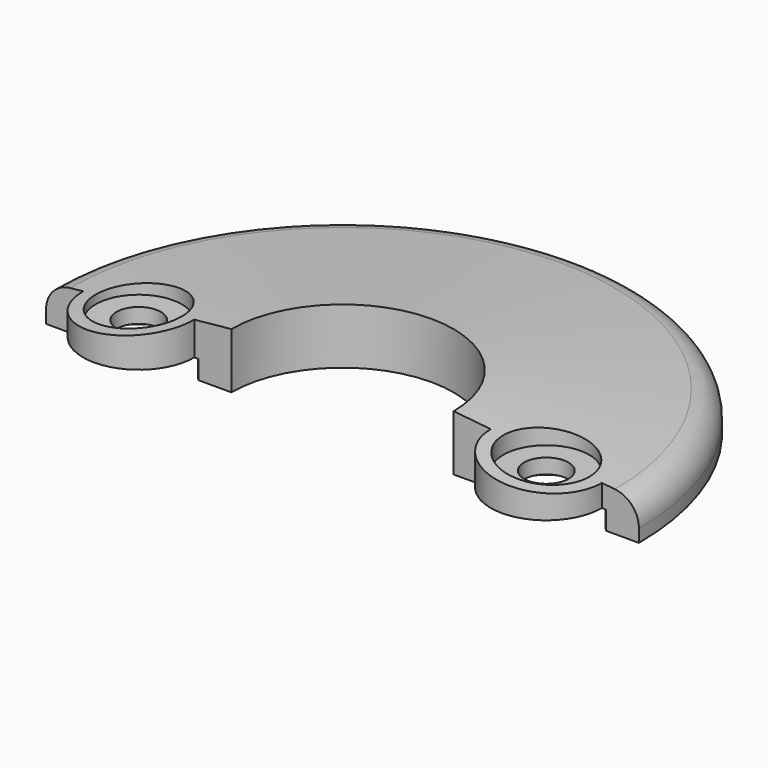
from build123d import *

# Parameters (mm, degrees)
F3_DEPTH     = 4.7762
F4_R         = 4.8895
F5_DEPTH     = 1.6002
F6_R         = 1.905
F7_DEPTH     = 3.1760001
F9_R         = 3.683
F10_DEPTH    = 1.9060001
F11_T1_DEPTH = 2.2381504403


# Not quite as in the source:
# - a fillet or chamfer that OpenCascade refuses, or shapes differently, is made with other operations: its cross-section is extruded or revolved along the edge and cut away or added


with BuildPart() as f1:
    # F0 (on Front) → F1 (revolve)
    with BuildSketch(Plane.XZ):
        with BuildLine():
            Line((9.525, 4.7752), (9.525, 0))
            Line((9.525, 0), (25.4, 0))
            Line((25.4, 0), (25.4, 1.10784454))
            ThreePointArc((25.4, 1.10784454), (24.8095678029, 2.6410913648), (23.343266994, 3.382318687))
            Line((23.343266994, 3.382318687), (9.525, 4.7752))
        make_face()
    revolve(axis=Axis((0, 0, 2.1961550228), (0, 0, 1)))

    # F2 (on face) → F3 (cut, through all)
    with BuildSketch(Plane(origin=(0, 0, 0), x_dir=(1, 0, 0), z_dir=(0, 0, -1))):
        with BuildLine():
            Line((-25.4, 25.4), (-25.4, 0))
            Line((-25.4, 0), (-22.225, 0))
            ThreePointArc((-22.225, 0), (-17.4625, 4.7625), (-12.7, 0))
            Line((-12.7, 0), (-9.525, 0))
            ThreePointArc((-9.525, 0), (0, 9.525), (9.525, 0))
            Line((9.525, 0), (12.7, 0))
            ThreePointArc((12.7, 0), (17.4625, 4.7625), (22.225, 0))
            Line((22.225, 0), (25.4, 0))
            Line((25.4, 0), (25.4, 25.4))
            Line((25.4, 25.4), (-25.4, 25.4))
        make_face()
        with BuildLine():
            ThreePointArc((9.525, 0), (0, 9.525), (-9.525, 0))
            ThreePointArc((-9.525, 0), (0, -9.525), (9.525, 0))
        make_face()
    extrude(amount=-F3_DEPTH, mode=Mode.SUBTRACT)

    # F4 (on face) → F5 (cut)
    with BuildSketch(Plane(origin=(0, 0, 0), x_dir=(1, 0, 0), z_dir=(0, 0, -1))):
        with Locations((-17.4625, 0)):
            Circle(F4_R)
        with Locations((17.4625, 0)):
            Circle(F4_R)
    extrude(amount=-F5_DEPTH, mode=Mode.SUBTRACT)

    # F6 (on face) → F7 (cut, through all)
    with BuildSketch(Plane(origin=(0, 0, 1.6002), x_dir=(1, 0, 0), z_dir=(0, 0, -1))):
        with Locations((-17.4625, 0)):
            Circle(F6_R)
        with Locations((17.4625, 0)):
            Circle(F6_R)
    extrude(amount=-F7_DEPTH, mode=Mode.SUBTRACT)

    # F9 (on offset) → F10 (cut, through all)
    with BuildSketch(Plane(origin=(0, 0, 2.8702), x_dir=(1, 0, 0), z_dir=(0, 0, -1))):
        with Locations((17.4625, 0)):
            Circle(F9_R)
        with Locations((-17.4625, 0)):
            Circle(F9_R)
    extrude(amount=-F10_DEPTH, mode=Mode.SUBTRACT)

    # F11: chamfer of 0.254 on 4 edges, made by hand

    # F11_s2 → F11_t1 (cut)
    with BuildSketch(Plane.XY.offset(-0.6379504403)):
        with BuildLine():
            Line((-22.3460344648, 0.2414567901), (-22.5997245668, 0))
            Line((-22.5997245668, 0), (-22.352, 0))
            ThreePointArc((-22.352, 0), (-22.3504182536, 0.1243599467), (-22.3460344648, 0.2414567901))
        make_face()
        with BuildLine():
            Line((-12.5789655352, 0.2414567901), (-12.3252754332, 0))
            Line((-12.3252754332, 0), (-12.573, 0))
            ThreePointArc((-12.573, 0), (-12.5745817464, 0.1243599467), (-12.5789655352, 0.2414567901))
        make_face()
        with BuildLine():
            Line((12.5789655352, 0.2414567901), (12.3252754332, 0))
            Line((12.3252754332, 0), (12.573, 0))
            ThreePointArc((12.573, 0), (12.5745817464, 0.1243599467), (12.5789655352, 0.2414567901))
        make_face()
        with BuildLine():
            Line((22.3460344648, 0.2414567901), (22.5997245668, 0))
            Line((22.5997245668, 0), (22.352, 0))
            ThreePointArc((22.352, 0), (22.3504182536, 0.1243599467), (22.3460344648, 0.2414567901))
        make_face()
    extrude(amount=F11_T1_DEPTH, mode=Mode.SUBTRACT)


solid = f1.part
